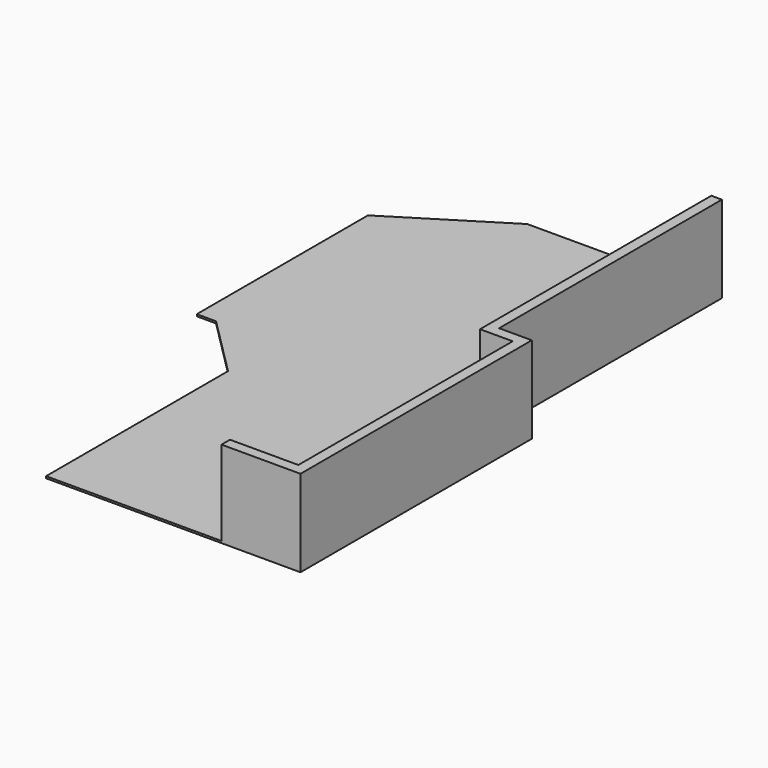
from build123d import *

# Parameters (mm, degrees)
F1_DEPTH = 25.4
F2_DEPTH = 1117.6


# Not quite as in the source:
# - the program builds the solid bodies; features that only make, move or delete a surface that nothing else refers to are left out


with BuildPart() as f1:
    # F0 (on Top) → F1 (new body)
    with BuildSketch(Plane.XY):
        Polygon((-1041.4, 0), (0, 0), (0, 3810), (-430.6243517664, 3810), (-430.6243517664, 7480.3), (-570.3243517664, 7480.3), (-570.3243517664, 3810), (-570.3243517664, 3670.3), (-139.7, 3670.3), (-139.7, 139.7), (-1041.4, 139.7), align=None)
        Polygon((-3352.8, 0), (-1041.4, 0), (-1041.4, 139.7), (-139.7, 139.7), (-139.7, 3670.3), (-570.3243517664, 3670.3), (-570.3243517664, 3810), (-570.3243517664, 7480.3), (-2996.0243517664, 7480.3), (-4397.0625386541, 6606.8625386541), (-4397.0625386541, 3787.4625386541), (-4143.0625386541, 3787.4625386541), (-3352.8, 2997.2), align=None)
    extrude(amount=-F1_DEPTH)

    # F0 (on Top) → F2 (join)
    with BuildSketch(Plane.XY):
        Polygon((-1041.4, 0), (0, 0), (0, 3810), (-430.6243517664, 3810), (-430.6243517664, 7480.3), (-570.3243517664, 7480.3), (-570.3243517664, 3810), (-570.3243517664, 3670.3), (-139.7, 3670.3), (-139.7, 139.7), (-1041.4, 139.7), align=None)
    extrude(amount=F2_DEPTH)


solid = f1.part
